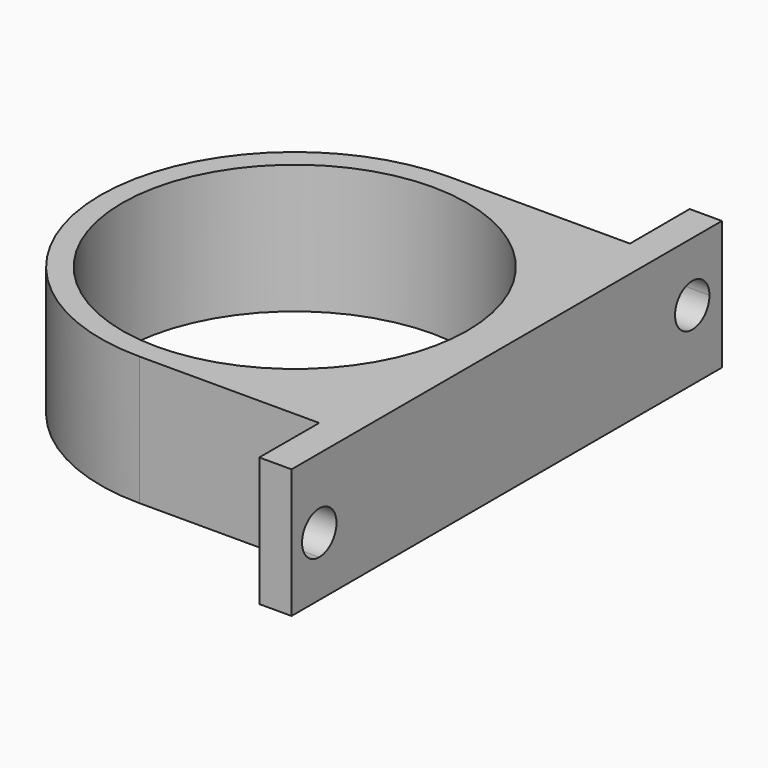
from build123d import *

# Parameters (mm, degrees)
F0_R     = 16.05
F1_DEPTH = 12
F3_DEPTH = 25
F5_DEPTH = 25


# Not quite as in the source:
# - a feature names something its author has since deleted; it is built from what else it names


with BuildPart() as f1:
    # F0 (on Top) → F1 (new body)
    with BuildSketch(Plane.XY):
        with BuildLine():
            ThreePointArc((0, -18.05), (12.7632774004, -12.7632774004), (18.05, 0))
            ThreePointArc((18.05, 0), (12.7632774004, 12.7632774004), (0, 18.05))
            ThreePointArc((0, 18.05), (-18.05, 0), (0, -18.05))
        make_face()
        Circle(F0_R, mode=Mode.SUBTRACT)
        with BuildLine():
            ThreePointArc((0, 18.05), (12.7632774004, 12.7632774004), (18.05, 0))
            ThreePointArc((18.05, 0), (12.7632774004, -12.7632774004), (0, -18.05))
            Line((0, -18.05), (16.7152378708, -18.05))
            Line((16.7152378708, -18.05), (16.7, -25))
            Line((16.7, -25), (19.7, -25))
            Line((19.7, -25), (19.7, 0))
            Line((19.7, 0), (19.7, 25))
            Line((19.7, 25), (16.7, 25))
            Line((16.7, 25), (16.7152378708, 18.05))
            Line((16.7152378708, 18.05), (0, 18.05))
        make_face()
    extrude(amount=F1_DEPTH)

    # F2 (on face) → F3 (cut)
    with BuildSketch(Plane(origin=(16.754731944, -0.0367347397, 0), x_dir=(-0.0021924941, -0.9999975965, 0), z_dir=(-0.9999975965, 0.0021924941, 0))):
        with BuildLine():
            ThreePointArc((23.7358004302, 5.5), (20.3215868678, 6.9142135624), (21.7358004302, 3.5))
            Line((21.7358004302, 3.5), (21.7358004302, 5.5))
            Line((21.7358004302, 5.5), (23.7358004302, 5.5))
        make_face()
        with BuildLine():
            Line((21.7358004302, 5.5), (21.7358004302, 3.5))
            ThreePointArc((21.7358004302, 3.5), (23.1500139926, 4.0857864376), (23.7358004302, 5.5))
            Line((23.7358004302, 5.5), (21.7358004302, 5.5))
        make_face()
    extrude(amount=-F3_DEPTH, mode=Mode.SUBTRACT)

    # F4 (on face) → F5 (cut)
    with BuildSketch(Plane(origin=(16.754731944, 0.0367347397, 0), x_dir=(0.0021924941, -0.9999975965, 0), z_dir=(-0.9999975965, -0.0021924941, 0))):
        with BuildLine():
            Line((-21.5104483068, 6.5), (-21.5104483068, 8.5))
            ThreePointArc((-21.5104483068, 8.5), (-22.9246618692, 7.9142135624), (-23.5104483068, 6.5))
            Line((-23.5104483068, 6.5), (-21.5104483068, 6.5))
        make_face()
        with BuildLine():
            ThreePointArc((-19.5104483068, 6.5), (-20.0962347444, 7.9142135624), (-21.5104483068, 8.5))
            Line((-21.5104483068, 8.5), (-21.5104483068, 6.5))
            Line((-21.5104483068, 6.5), (-23.5104483068, 6.5))
            ThreePointArc((-23.5104483068, 6.5), (-21.5104483068, 4.5), (-19.5104483068, 6.5))
        make_face()
    extrude(amount=-F5_DEPTH, mode=Mode.SUBTRACT)


solid = f1.part
